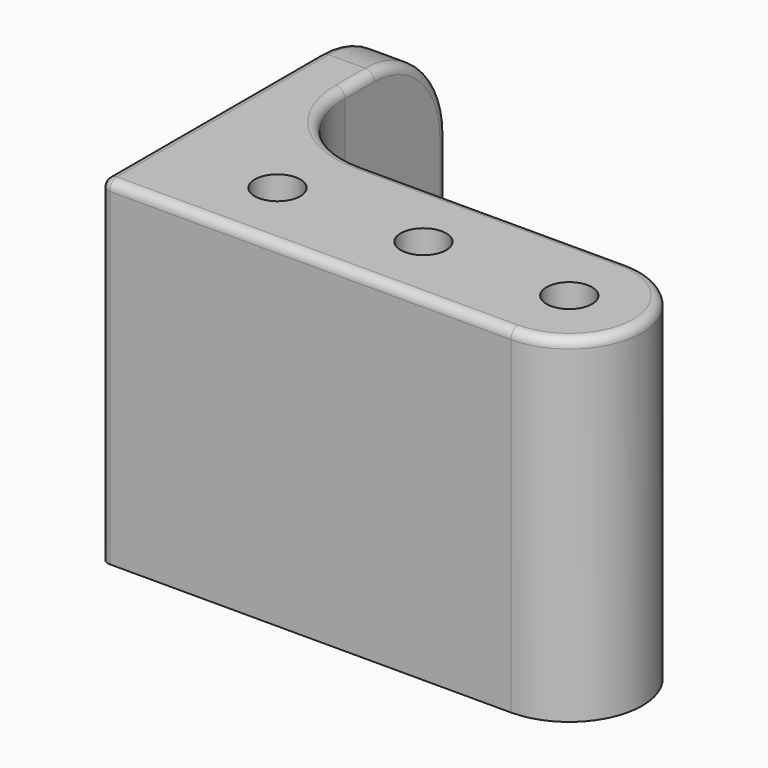
from build123d import *

# Parameters (mm, degrees)
F0_R           = 1.5
F1_DEPTH       = 18.5
F2_D           = 2.5
F3_D           = 2.5
F3_CSINK_D     = 6.72
F3_CSINK_ANGLE = 90
F4_R           = 5
F5_R           = 0.5


with BuildPart() as f1:
    # F0 (on Top) → F1 (new body)
    with BuildSketch(Plane.XY):
        with BuildLine():
            Line((-14.5, -4), (8, -4))
            ThreePointArc((8, -4), (12, 0), (8, 4))
            Line((8, 4), (-11.5, 4))
            Line((-11.5, 4), (-11.5, 16))
            Line((-11.5, 16), (-14.5, 16))
            Line((-14.5, 16), (-14.5, -4))
        make_face()
        with Locations((-8, 0)):
            Circle(F0_R, mode=Mode.SUBTRACT)
        Circle(F0_R, mode=Mode.SUBTRACT)
        with Locations((8, 0)):
            Circle(F0_R, mode=Mode.SUBTRACT)
        Circle(F0_R)
        with Locations((8, 0)):
            Circle(F0_R)
        with Locations((-8, 0)):
            Circle(F0_R)
    extrude(amount=F1_DEPTH)

    # F2 (through all)
    with Locations(Plane(origin=(0, 0, 0), x_dir=(1, 0, 0), z_dir=(0, 0, -1))):
        with Locations((8, 0), (0, 0)):
            Hole(F2_D / 2)

    # F3 (through all)
    with Locations(Plane(origin=(0, 0, 0), x_dir=(1, 0, 0), z_dir=(0, 0, -1))):
        with Locations((-8, 0)):
            CounterSinkHole(F3_D / 2, F3_CSINK_D / 2, counter_sink_angle=F3_CSINK_ANGLE)

    # F4
    f4_edges = [f1.edges().sort_by_distance(p)[0] for p in [
        (-11.5, 4, 9.25),
        (-13, 16, 18.5),
    ]]
    fillet(f4_edges, radius=F4_R)

    # F5
    f5_edges = [f1.edges().sort_by_distance(p)[0] for p in [
        (-3.25, -4, 18.5),
        (-14.5, 3.5, 18.5),
        (-14.5, 14.535534, 17.035534),
        (-14.5, -4, 9.25),
    ]]
    fillet(f5_edges, radius=F5_R)


solid = f1.part
